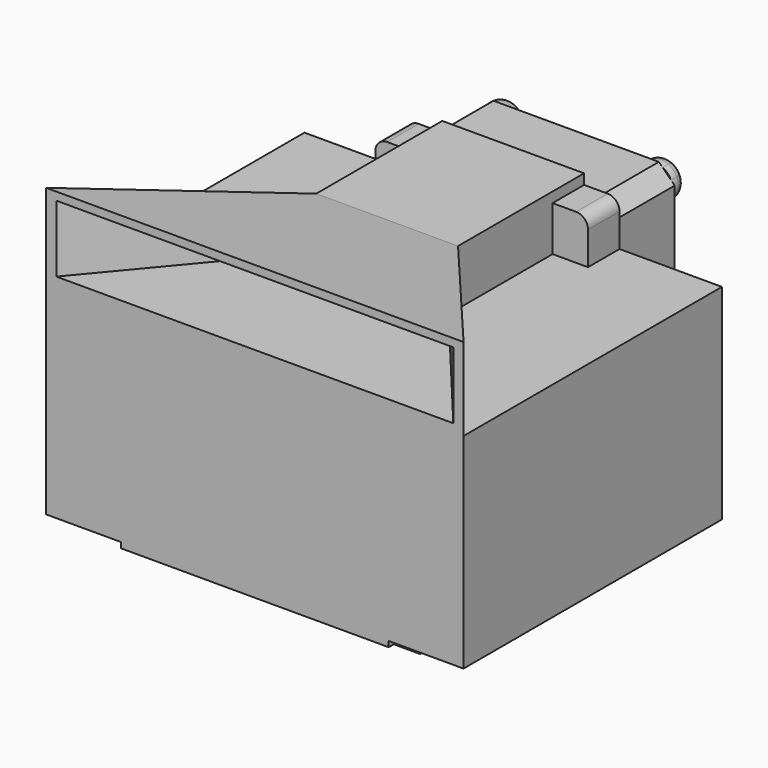
from build123d import *

# Parameters (mm, degrees)
F0_W      = 53
F0_H      = 26
F1_DEPTH  = 41
F2_W      = 18
F2_H      = 20
F3_DEPTH  = 7
F3_FACE_W = 18
F3_FACE_H = 7
F4_W      = 53
F4_H      = 10.5
F6_T      = -1
F7_W      = 34
F7_H      = 5
F8_DEPTH  = 0.7
F7_H_2    = 36
F9_DEPTH  = 3.5
F10_W     = 3.5
F10_H     = 4.7
F11_DEPTH = 10
F12_SIZE  = 2
F13_DEPTH = 5
F14_R     = 1.5
F16_DEPTH = 2
F17_R     = 1.1
F18_W     = 7.5
F18_H     = 1
F19_DEPTH = 12
F20_R     = 0.49999


# Not quite as in the source:
# - a fillet or chamfer is up to 0.001 mm smaller than in the source, because OpenCascade refuses the exact size
# - a feature names something its author has since deleted; it is built from what else it names


with BuildPart() as f1:
    # F0 (on Front) → F1 (new body)
    with BuildSketch(Plane.XZ):
        Rectangle(F0_W, F0_H)
    extrude(amount=-F1_DEPTH)

    # F2 (on face) → F3 (join)
    with BuildSketch(Plane.XY.offset(13)):
        with Locations((0, 31)):
            Rectangle(F2_W, F2_H)
    extrude(amount=F3_DEPTH)



with BuildPart() as f5:
    # F3_face (on face) → F5 section 0
    with BuildSketch(Plane(origin=(0, 21, 16.5), x_dir=(1, 0, 0), z_dir=(0, -1, 0))):
        Rectangle(F3_FACE_W, F3_FACE_H)
    # F4 (on face) → F5 section 1
    with BuildSketch(Plane.XZ):
        with Locations((0, 18.25)):
            Rectangle(F4_W, F4_H)
    loft()

    # F6
    f6_openings = [f5.faces().sort_by_distance(p)[0] for p in [
        (0, 0, 18.25),
    ]]
    offset(amount=F6_T, openings=f6_openings)


with BuildPart() as f1_1:
    add(f1.part)

    add(f5.part)  # F8 merges F5
    # F7 (on face) → F8 (join)
    with BuildSketch(Plane(origin=(0, 0, -13), x_dir=(1, 0, 0), z_dir=(0, 0, -1))):
        with Locations((0, -2.5)):
            Rectangle(F7_W, F7_H)
    extrude(amount=F8_DEPTH)

    # F7 (on face) → F9 (join)
    with BuildSketch(Plane(origin=(0, 0, -13), x_dir=(1, 0, 0), z_dir=(0, 0, -1))):
        with Locations((0, -23)):
            Rectangle(F7_W, F7_H_2)
    extrude(amount=F9_DEPTH)

    # F10 (on face) → F11 (join)
    with BuildSketch(Plane(origin=(0, 41, 0), x_dir=(-1, 0, 0), z_dir=(0, 1, 0))):
        with Locations((10.75, 15.35)):
            Rectangle(F10_W, F10_H)
        Polygon((9, 17.7), (-9, 17.7), (-9, 13), (-12.5, 13), (-12.5, -7.3), (12.5, -7.3), (12.5, 13), (9, 13), align=None)
        with Locations((-10.75, 15.35)):
            Rectangle(F10_W, F10_H)
    extrude(amount=F11_DEPTH)

    # F12
    f12_edges = [f1_1.edges().sort_by_distance(p)[0] for p in [
        (12.5, 46, 17.7),
        (-12.5, 46, 17.7),
        (-12.5, 46, -7.3),
        (12.5, 46, -7.3),
    ]]
    chamfer(f12_edges, length=F12_SIZE)

    # F10 (on face) → F13 (join)
    with BuildSketch(Plane(origin=(0, 41, 0), x_dir=(-1, 0, 0), z_dir=(0, 1, 0))):
        Polygon((-12.5, 13), (-12.5, 17.7), (-9, 17.7), (-9, 18.6999991059), (-13.4999991059, 18.6999991059), (-13.4999991059, 13), align=None)
        with Locations((-10.75, 15.35)):
            Rectangle(F10_W, F10_H)
        Polygon((9, 18.6999991059), (9, 17.7), (12.5, 17.7), (12.5, 13), (13.4999991059, 13), (13.4999991059, 18.6999991059), align=None)
        with Locations((10.75, 15.35)):
            Rectangle(F10_W, F10_H)
    extrude(amount=-F13_DEPTH)

    # F14
    f14_edges = [f1_1.edges().sort_by_distance(p)[0] for p in [
        (13.499999, 38.5, 18.699999),
        (-13.499999, 38.5, 18.699999),
    ]]
    fillet(f14_edges, radius=F14_R)

    # F15 (on face) → F16 (join)
    with BuildSketch(Plane(origin=(0, 51, 0), x_dir=(-1, 0, 0), z_dir=(0, 1, 0))):
        with BuildLine():
            ThreePointArc((-12.0303300859, 16.1696699141), (-10.4971203611, 13.0056045601), (-7.75, 15.2))
            ThreePointArc((-7.75, 15.2), (-8.7998452822, 17.1031890745), (-10.9696699141, 17.2303300859))
            Line((-10.9696699141, 17.2303300859), (-12.0303300859, 16.1696699141))
        make_face()
        with BuildLine():
            ThreePointArc((12.0303300859, 16.1696699141), (11.5909902577, 16.7909902577), (10.9696699141, 17.2303300859))
            Line((10.9696699141, 17.2303300859), (12.0303300859, 16.1696699141))
        make_face()
        with BuildLine():
            Line((10.9696699141, -6.8303300859), (12.0303300859, -5.7696699141))
            ThreePointArc((12.0303300859, -5.7696699141), (12.1943954399, -5.2971203611), (12.25, -4.8))
            ThreePointArc((12.25, -4.8), (8.0968109255, -3.5998452822), (10.9696699141, -6.8303300859))
        make_face()
        with BuildLine():
            Line((-10.9696699141, -6.8303300859), (-12.0303300859, -5.7696699141))
            ThreePointArc((-12.0303300859, -5.7696699141), (-11.5909902577, -6.3909902577), (-10.9696699141, -6.8303300859))
        make_face()
        with BuildLine():
            Line((-12.0303300859, 16.1696699141), (-10.9696699141, 17.2303300859))
            ThreePointArc((-10.9696699141, 17.2303300859), (-11.5909902577, 16.7909902577), (-12.0303300859, 16.1696699141))
        make_face()
        with BuildLine():
            ThreePointArc((-7.75, -4.8), (-10.4971203611, -2.6056045601), (-12.0303300859, -5.7696699141))
            Line((-12.0303300859, -5.7696699141), (-10.9696699141, -6.8303300859))
            ThreePointArc((-10.9696699141, -6.8303300859), (-8.7998452822, -6.7031890745), (-7.75, -4.8))
        make_face()
        with BuildLine():
            ThreePointArc((10.9696699141, -6.8303300859), (11.5909902577, -6.3909902577), (12.0303300859, -5.7696699141))
            Line((12.0303300859, -5.7696699141), (10.9696699141, -6.8303300859))
        make_face()
        with BuildLine():
            Line((12.0303300859, 16.1696699141), (10.9696699141, 17.2303300859))
            ThreePointArc((10.9696699141, 17.2303300859), (8.0968109255, 13.9998452822), (12.25, 15.2))
            ThreePointArc((12.25, 15.2), (12.1943954399, 15.6971203611), (12.0303300859, 16.1696699141))
        make_face()
    extrude(amount=F16_DEPTH)

    # F17
    f17_edges = [f1_1.edges().sort_by_distance(p)[0] for p in [
        (9.03033, 53, 13.16967),
        (-9.03033, 53, 13.16967),
        (9.03033, 53, -2.76967),
        (-9.03033, 53, -2.76967),
    ]]
    fillet(f17_edges, radius=F17_R)

    # F18 (on face) → F19 (join)
    with BuildSketch(Plane(origin=(-17, 0, 0), x_dir=(0, -1, 0), z_dir=(-1, 0, 0))):
        with Locations((-19.75, -13.5)):
            Rectangle(F18_W, F18_H)
    extrude(amount=F19_DEPTH)

    # F20 (radius 0.5 in the source; OpenCascade refuses exactly that, so slightly less here)
    f20_edges = [f1_1.edges().sort_by_distance(p)[0] for p in [
        (-23, 16, -14),
        (-27.75, 16, -13),
        (-23, 23.5, -14),
        (-27.75, 23.5, -13),
    ]]
    fillet(f20_edges, radius=F20_R)


solid = f1_1.part
